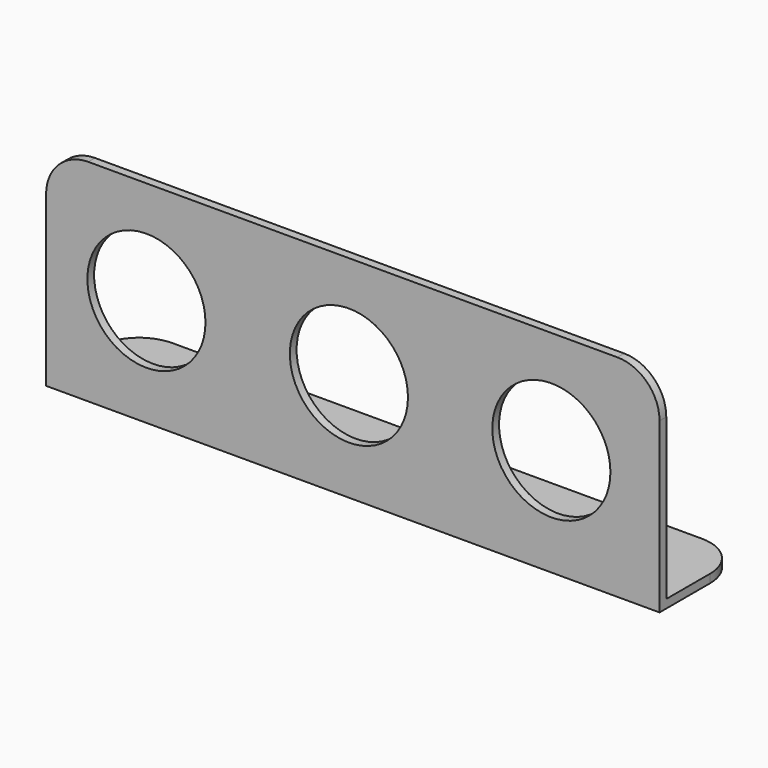
from build123d import *

# Parameters (mm, degrees)
F0_W     = 145.4322189093
F0_H     = 48
F0_R     = 14
F1_DEPTH = 2
F3_R     = 10
F4_W     = 145.4322189093
F4_H     = 25
F5_DEPTH = 2
F6_R     = 10


with BuildPart() as f1:
    # F0 (on Front) → F1 (new body)
    with BuildSketch(Plane.XZ):
        with Locations((0.9282901883, 0.5)):
            Rectangle(F0_W, F0_H)
        with Locations((-48, 0)):
            Circle(F0_R, mode=Mode.SUBTRACT)
        Circle(F0_R, mode=Mode.SUBTRACT)
        with Locations((48, 0)):
            Circle(F0_R, mode=Mode.SUBTRACT)
    extrude(amount=F1_DEPTH)

    # F3
    f3_edges = [f1.edges().sort_by_distance(p)[0] for p in [
        (73.6444, -1, 24.5),
        (-71.787819, -1, 24.5),
    ]]
    fillet(f3_edges, radius=F3_R)

    # F4 (on offset) → F5 (join)
    with BuildSketch(Plane(origin=(0, 0, -23.5), x_dir=(1, 0, 0), z_dir=(0, 0, -1))):
        with Locations((0.9282901883, -10.5)):
            Rectangle(F4_W, F4_H)
    extrude(amount=F5_DEPTH)

    # F6
    f6_edges = [f1.edges().sort_by_distance(p)[0] for p in [
        (-71.787819, 23, -24.5),
        (73.6444, 23, -24.5),
    ]]
    fillet(f6_edges, radius=F6_R)


solid = f1.part
